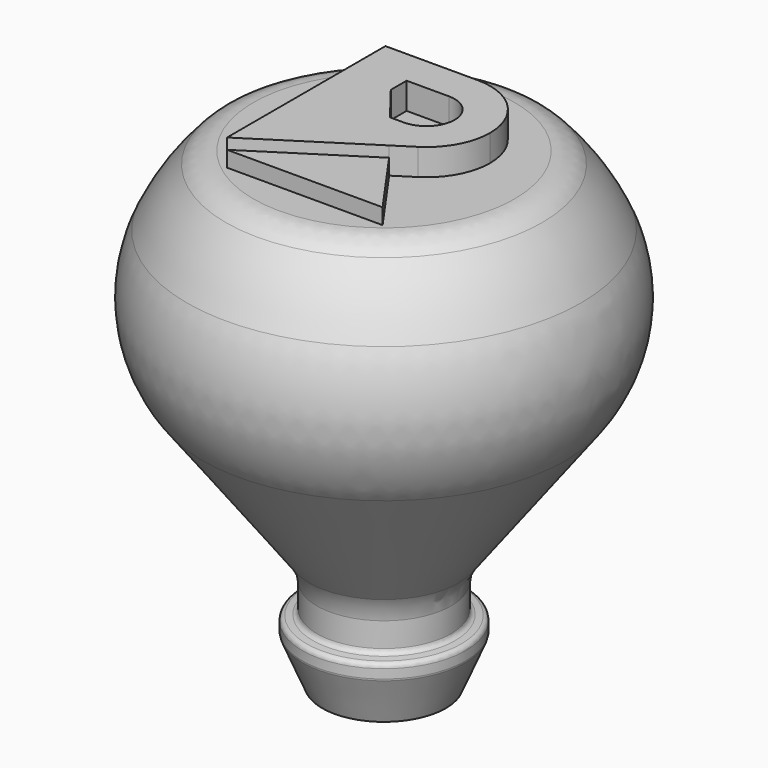
from build123d import *

# Parameters (mm, degrees)
F2_R     = 19.05
F3_R     = 5.08
F4_R     = 0.635
F5_R     = 5.08
F7_START = 62.40395
F7_DEPTH = 3.00105
F8_START = 62.38159
F8_DEPTH = 2.05007
F9_SCALE = 1.5


with BuildPart() as f1:
    # F0 (on Front) → F1 (revolve)
    with BuildSketch(Plane.XZ):
        with BuildLine():
            Line((8.3312, 0), (10.9982, 6.35))
            Line((10.9982, 6.35), (10.9982, 8.255))
            Line((10.9982, 8.255), (9.0424, 8.509))
            Line((9.0424, 8.509), (9.0424, 14.0462))
            Line((9.0424, 14.0462), (29.196018501, 40.9176913346))
            ThreePointArc((29.196018501, 40.9176913346), (26.8994300075, 53.2075181262), (19.6747553987, 63.4113526052))
            Line((19.6747553987, 63.4113526052), (0, 63.4113526052))
            Line((0, 63.4113526052), (0, 61.087))
            Line((0, 61.087), (1.9812, 61.087))
            Line((1.9812, 61.087), (4.5212, 58.547))
            Line((4.5212, 58.547), (4.5212, 33.147))
            Line((4.5212, 33.147), (7.0612, 28.067))
            Line((7.0612, 28.067), (7.0612, 0))
            Line((7.0612, 0), (8.3312, 0))
        make_face()
    revolve(axis=Axis((0, 0, 62.2491763026), (0, 0, 1)))

    # F2
    f2_edges = [f1.edges().sort_by_distance(p)[0] for p in [
        (-29.196019, 0, 40.917691),
    ]]
    fillet(f2_edges, radius=F2_R)

    # F3
    f3_edges = [f1.edges().sort_by_distance(p)[0] for p in [
        (-19.674755, 0, 63.411353),
    ]]
    fillet(f3_edges, radius=F3_R)

    # F4
    f4_edges = [f1.edges().sort_by_distance(p)[0] for p in [
        (-10.9982, 0, 8.255),
        (-10.9982, 0, 6.35),
        (-9.0424, 0, 8.509),
    ]]
    fillet(f4_edges, radius=F4_R)

    # F5
    f5_edges = [f1.edges().sort_by_distance(p)[0] for p in [
        (-9.0424, 0, 14.0462),
    ]]
    fillet(f5_edges, radius=F5_R)


with BuildPart() as f7:
    # F6 (on Top) → F7 (new body)
    with BuildSketch(Plane.XY.offset(F7_START)):
        with BuildLine():
            ThreePointArc((6.985, 3.1749999976), (5.3111152553, 7.2161152536), (1.27, 8.89))
            Line((1.27, 8.89), (-6.985, 8.89))
            Line((-6.985, 8.89), (-6.985, -8.89))
            Line((-6.985, -8.89), (2.6434823599, -2.7306796279))
            Line((2.6434823599, -2.7306796279), (4.349660186, -1.6392411799))
            ThreePointArc((4.349660186, -1.6392411799), (6.2830570988, 0.4308273516), (6.985, 3.1749999976))
        make_face()
        with BuildLine():
            ThreePointArc((1.2915025508, 0.6350910173), (1.27, 0.635), (1.2484974492, 0.6350910173))
            Line((1.2484974492, 0.6350910173), (0.0272060427, 0.6350910173))
            Line((0.0272060427, 0.6350910173), (-2.54, 3.9377340455))
            Line((-2.54, 3.9377340455), (-2.54, 5.715))
            Line((-2.54, 5.715), (1.27, 5.715))
            ThreePointArc((1.27, 5.715), (3.8099772456, 3.1857513717), (1.2915025508, 0.6350910173))
        make_face(mode=Mode.SUBTRACT)
    extrude(amount=F7_DEPTH)

    # F6 (on Top) → F8 (join)
    with BuildSketch(Plane.XY.offset(F8_START)):
        Polygon((2.6434823599, -2.7306796279), (-6.985, -8.89), (6.985, -8.89), align=None)
    extrude(amount=F8_DEPTH)


with BuildPart() as f7_1:
    # F9: moved
    add(f7.part.scale(F9_SCALE))


with BuildPart() as f7_2:
    # F10: moved
    add(f7_1.part.moved(Location((0, 0, -31.115))))


solid = Compound([f1.part, f7_2.part])
